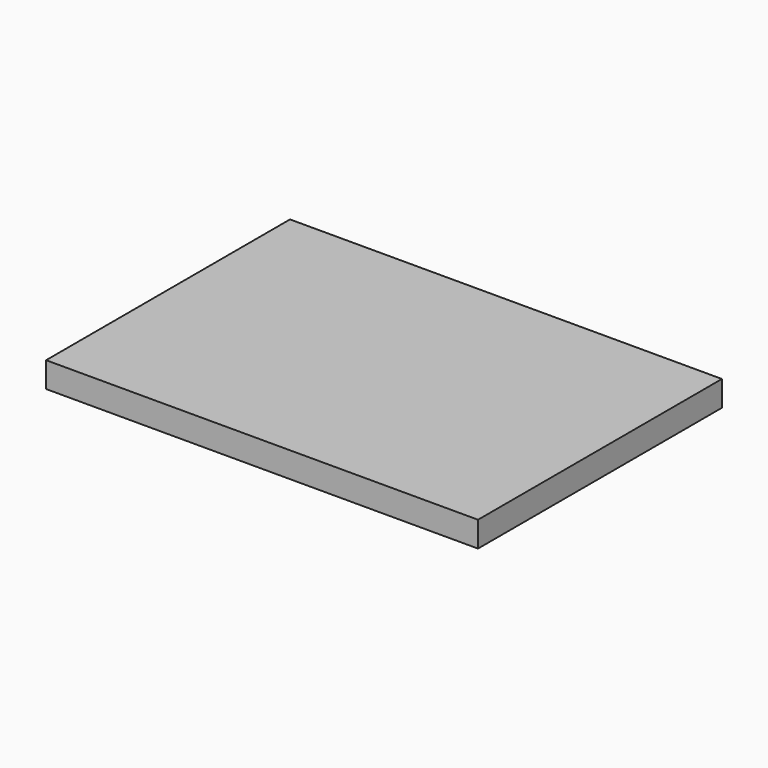
from build123d import *

# Parameters (mm, degrees)
F0_W     = 170
F0_H     = 120
F1_DEPTH = 10


# Not quite as in the source:
# - a feature names something its author has since deleted; it is built from what else it names


with BuildPart() as f1:
    # F0 (on Top) → F1 (new body)
    with BuildSketch(Plane.XY):
        Rectangle(F0_W, F0_H)
    extrude(amount=F1_DEPTH)


solid = f1.part
